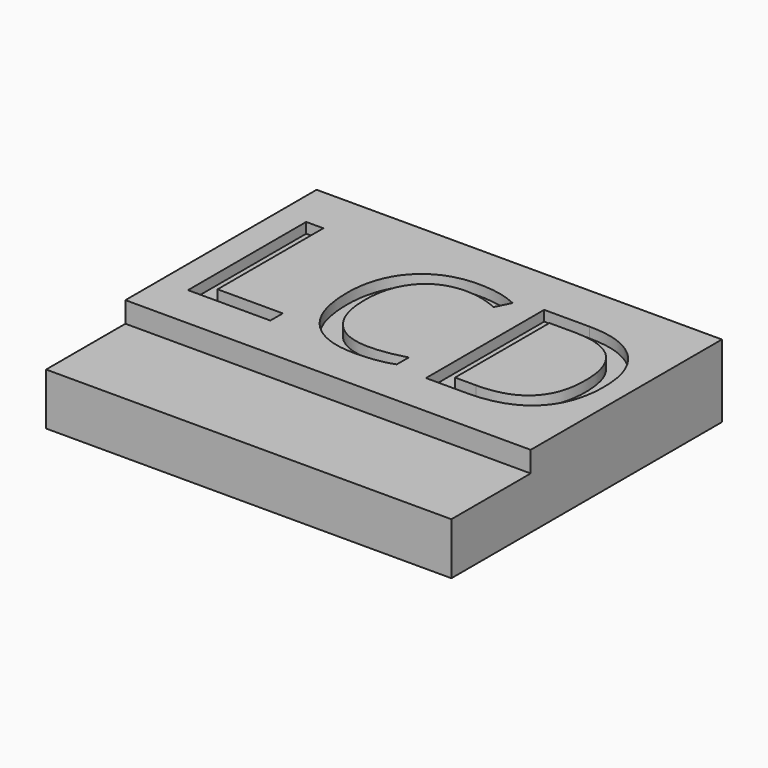
from build123d import *

# Parameters (mm, degrees)
F0_W         = 39
F0_H         = 9.54
F0_H_2       = 23
F1_DEPTH     = 5
F2_W         = 39
F2_H         = 23
F3_DEPTH     = 2
F4_TEXT_SIZE = 19.9133368571
F5_DEPTH     = 1


# Not quite as in the source:
# - Text() gives the source's letters only with a copy of the font that has no kerning and outlines rounded to 1/6400 em; it was checked with that copy


with BuildPart() as f1:
    # F0 (on Top) → F1 (new body)
    with BuildSketch(Plane.XY):
        with Locations((10.9838716984, -14.2824198115)):
            Rectangle(F0_W, F0_H)
        with Locations((10.9838716984, 1.9875801885)):
            Rectangle(F0_W, F0_H_2)
    extrude(amount=F1_DEPTH)

    # F2 (on face) → F3 (join)
    with BuildSketch(Plane.XY.offset(5)):
        with Locations((10.9838716984, 1.9875801885)):
            Rectangle(F2_W, F2_H)
    extrude(amount=F3_DEPTH)

    # F4 (on face) → F5 (cut)
    with BuildSketch(Plane.XY.offset(7)):
        with Locations((-7.8122145496, -5.3069777787)):
            Text('LCD', F4_TEXT_SIZE, font='Open Sans', text_align=(TextAlign.LEFT, TextAlign.BOTTOM))
    extrude(amount=-F5_DEPTH, mode=Mode.SUBTRACT)


solid = f1.part
